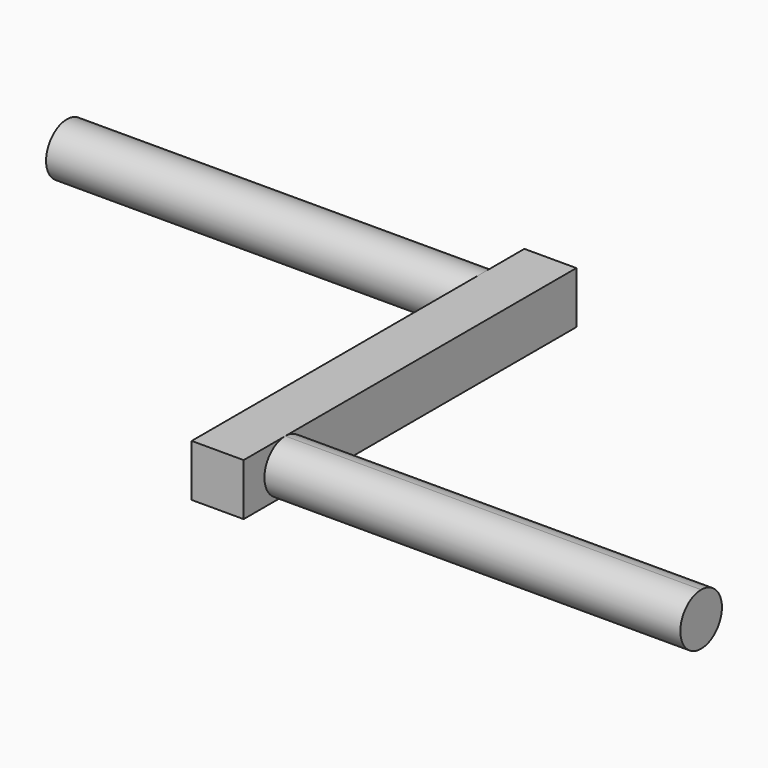
from build123d import *

# Parameters (mm, degrees)
F0_W     = 6.35
F0_H     = 6.35
F1_DEPTH = 25.4
F3_DEPTH = 50.8
F4_R     = 3.175
F5_DEPTH = 50.8


with BuildPart() as f1:
    # F0 (on Front) → F1 (new body, symmetric)
    with BuildSketch(Plane.XZ):
        Rectangle(F0_W, F0_H)
    extrude(amount=F1_DEPTH, both=True)

    # F2 (on face) → F3 (join)
    with BuildSketch(Plane.YZ.offset(3.175)):
        with BuildLine():
            ThreePointArc((-19.05, -3.175), (-16.8049359697, -2.2450640303), (-15.875, 0))
            ThreePointArc((-15.875, 0), (-16.8049359657, 2.2450640262), (-19.0499999885, 3.175))
            ThreePointArc((-19.0499999885, 3.175), (-22.225, 5.7e-09), (-19.05, -3.175))
        make_face()
    extrude(amount=F3_DEPTH)

    # F4 (on face) → F5 (join)
    with BuildSketch(Plane(origin=(-3.175, 0, 0), x_dir=(0, -1, 0), z_dir=(-1, 0, 0))):
        with Locations((-19.05, 0)):
            Circle(F4_R)
    extrude(amount=F5_DEPTH)


solid = f1.part
